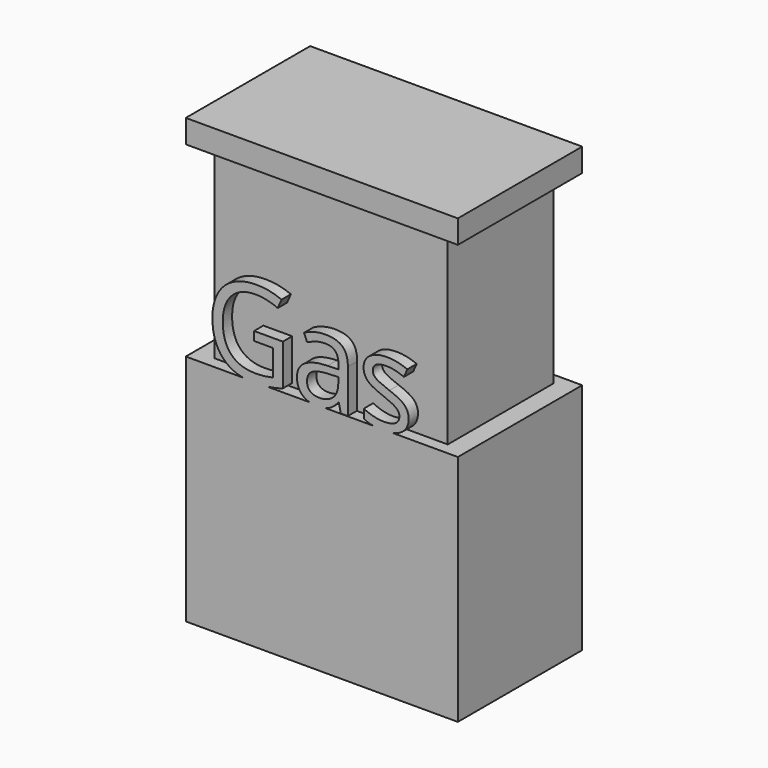
from build123d import *

# Parameters (mm, degrees)
F0_W         = 88.9
F0_H         = 50.8
F0_W_2       = 76.2
F0_H_2       = 43.18
F1_DEPTH     = 76.2
F2_DEPTH     = 140.97
F3_W         = 88.9
F3_H         = 7.62
F4_DEPTH     = 25.4
F3_TEXT_SIZE = 38.7666850454
F5_DEPTH     = 25.4


# Not quite as in the source:
# - the program builds the solid bodies; features that only make, move or delete a surface that nothing else refers to are left out
# - Text() gives the source's letters only with a copy of the font that has no kerning and outlines rounded to 1/6400 em; it was checked with that copy


with BuildPart() as f1:
    # F0 (on Top) → F1 (new body)
    with BuildSketch(Plane.XY):
        Rectangle(F0_W, F0_H)
        Rectangle(F0_W_2, F0_H_2, mode=Mode.SUBTRACT)
    extrude(amount=F1_DEPTH)

    # F0 (on Top) → F2 (join)
    with BuildSketch(Plane.XY):
        Rectangle(F0_W_2, F0_H_2)
    extrude(amount=F2_DEPTH)

    # F3 (on Front) → F4 (join, symmetric)
    with BuildSketch(Plane.XZ):
        with Locations((0, 141.032576561)):
            Rectangle(F3_W, F3_H)
    extrude(amount=F4_DEPTH, both=True)

    # F3 (on Front) → F5 (join)
    with BuildSketch(Plane.XZ):
        with Locations((0, 141.032576561)):
            Rectangle(F3_W, F3_H)
        with Locations((-38.1220020354, 76.2975737453)):
            Text('Gas', F3_TEXT_SIZE, font='Open Sans', text_align=(TextAlign.LEFT, TextAlign.BOTTOM))
    extrude(amount=F5_DEPTH)


solid = f1.part
